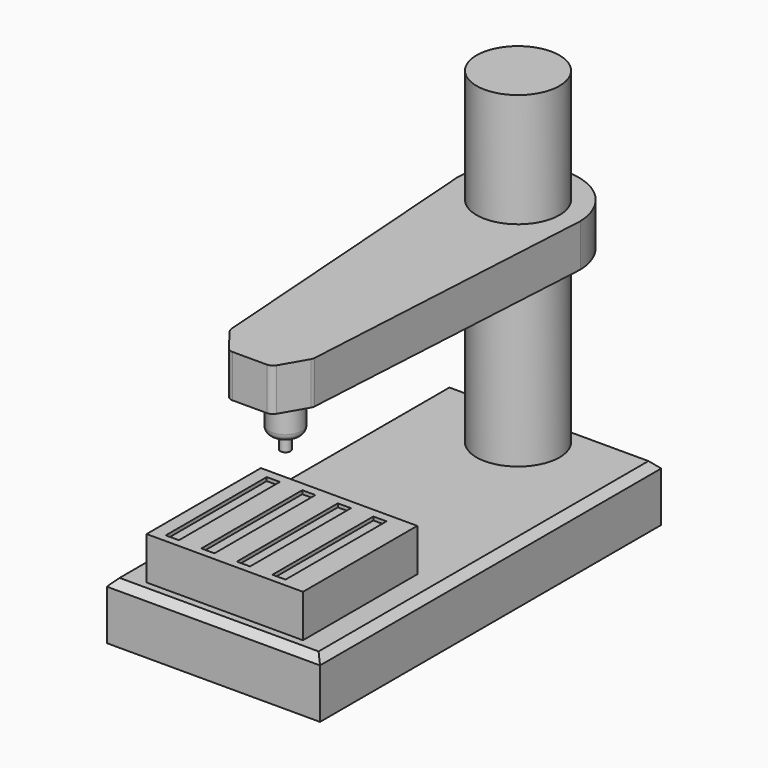
from build123d import *

# Parameters (mm, degrees)
F0_W          = 1500
F0_H          = 3000
F1_DEPTH      = 400
F2_R          = 292.2823500565
F3_DEPTH      = 1500
F4_W          = 1100
F4_H          = 1004.8507809427
F5_DEPTH      = 300
F6_W          = 92.4705266953
F6_H          = 887.717038393
F7_DEPTH      = 25
F9_DEPTH      = 300
F10_R         = 115.3363260379
F11_DEPTH     = 300
F12_R         = 50
F13_R         = 36.4638211497
F14_DEPTH     = 100
F15_T1_DEPTH  = 3257.1682987966
F15_T3_DEPTH  = 1757.1682987966
F15_T8_DEPTH  = 1757.1682987966
F15_S9_R      = 292.2823500565
F15_T10_DEPTH = 881
F16_R         = 55
F17_R         = 291.60933864
F18_DEPTH     = 800


# Not quite as in the source:
# - a fillet or chamfer that OpenCascade refuses, or shapes differently, is made with other operations: its cross-section is extruded or revolved along the edge and cut away or added


with BuildPart() as f1:
    # F0 (on Top) → F1 (new body)
    with BuildSketch(Plane.XY):
        with Locations((0.6129965186, 886.8090430593)):
            Rectangle(F0_W, F0_H)
    extrude(amount=F1_DEPTH)

    # F2 (on face) → F3 (join)
    with BuildSketch(Plane.XY.offset(400)):
        with Locations((0, 2065.9244060516)):
            Circle(F2_R)
    extrude(amount=F3_DEPTH)

    # F8 (on face) → F9 (join)
    with BuildSketch(Plane.XY.offset(1900)):
        with BuildLine():
            ThreePointArc((426.5312004435, 2082.0133865738), (-9.4648371748, 2492.653989164), (-426.8250972731, 2063.0859938416))
            Line((-426.8250972731, 2063.0859938416), (-269.5226555892, -131.283150546))
            Line((-269.5226555892, -131.283150546), (-120.9565666461, -326.7648934487))
            Line((-120.9565666461, -326.7648934487), (179.0434333539, -326.7648934487))
            Line((179.0434333539, -326.7648934487), (302.4182868002, -114.4829108661))
            Line((302.4182868002, -114.4829108661), (426.5312004435, 2082.0133865738))
        make_face()
    extrude(amount=-F9_DEPTH)

    # F10 (on face) → F11 (join)
    with BuildSketch(Plane(origin=(0, 0, 1600), x_dir=(1, 0, 0), z_dir=(0, 0, -1))):
        with Locations((16.4773444108, 0)):
            Circle(F10_R)
    extrude(amount=F11_DEPTH)

    # F12
    f12_edges = [f1.edges().sort_by_distance(p)[0] for p in [
        (-98.858982, 0, 1300),
    ]]
    fillet(f12_edges, radius=F12_R)

    # F13 (on face) → F14 (join)
    with BuildSketch(Plane(origin=(0, 0, 1300), x_dir=(1, 0, 0), z_dir=(0, 0, -1))):
        with Locations((16.4773444108, 0)):
            Circle(F13_R)
    extrude(amount=F14_DEPTH)

    # F15: chamfer of 50 on 4 edges, made by hand

    # F15_s2 → F15_t1 (cut)
    with BuildSketch(Plane.XZ.offset(-2515.3931924576)):
        Polygon((700.6129965186, 400), (750.6129965186, 350), (750.6129965186, 400), align=None)
        Polygon((-699.3870034814, 400), (-749.3870034814, 350), (-749.3870034814, 400), align=None)
    extrude(amount=F15_T1_DEPTH, mode=Mode.SUBTRACT)

    # F15_s4 → F15_t3 (cut)
    with BuildSketch(Plane.YZ.offset(-877.9711528797)):
        Polygon((-563.1909569407, 400), (-613.1909569407, 350), (-613.1909569407, 400), align=None)
    extrude(amount=F15_T3_DEPTH, mode=Mode.SUBTRACT)


with BuildPart() as f5:
    # F4 (on face) → F5 (new body)
    with BuildSketch(Plane.XY.offset(400)):
        with Locations((0.6129965186, -10.7655664693)):
            Rectangle(F4_W, F4_H)
    extrude(amount=F5_DEPTH)

    # F6 (on face) → F7 (cut)
    with BuildSketch(Plane.XY.offset(700)):
        with Locations((-411.1327528954, -15.5441612005)):
            Rectangle(F6_W, F6_H)
        with Locations((-161.1327528954, -15.5441612005)):
            Rectangle(F6_W, F6_H)
        with Locations((88.8672471046, -15.5441612005)):
            Rectangle(F6_W, F6_H)
        with Locations((338.8672471046, -15.5441612005)):
            Rectangle(F6_W, F6_H)
    extrude(amount=-F7_DEPTH, mode=Mode.SUBTRACT)


with BuildPart() as f15_tool6:
    # F15_s7 → F15_t8 (new body)
    with BuildSketch(Plane.YZ.offset(879.1971459169)):
        Polygon((2336.8090430593, 400), (2386.8090430593, 350), (2386.8090430593, 400), align=None)
    extrude(amount=-F15_T8_DEPTH)

    # F15_s9 → F15_t10 (cut, symmetric)
    with BuildSketch(Plane.XY.offset(375)):
        with Locations((0, 2065.9244060516)):
            Circle(F15_S9_R)
    extrude(amount=F15_T10_DEPTH, both=True, mode=Mode.SUBTRACT)


with BuildPart() as f1_1:
    add(f1.part)

    # F15_t5: cut F15_tool6
    add(f15_tool6.part, mode=Mode.SUBTRACT)

    # F16
    f16_edges = [f1_1.edges().sort_by_distance(p)[0] for p in [
        (302.418287, -114.482911, 1750),
        (179.043433, -326.764893, 1750),
        (-120.956567, -326.764893, 1750),
        (-269.522656, -131.283151, 1750),
    ]]
    fillet(f16_edges, radius=F16_R)

    # F17 (on face) → F18 (join)
    with BuildSketch(Plane.XY.offset(1900)):
        with Locations((0, 2065.9244060516)):
            Circle(F17_R)
    extrude(amount=F18_DEPTH)


solid = Compound([f5.part, f1_1.part])
